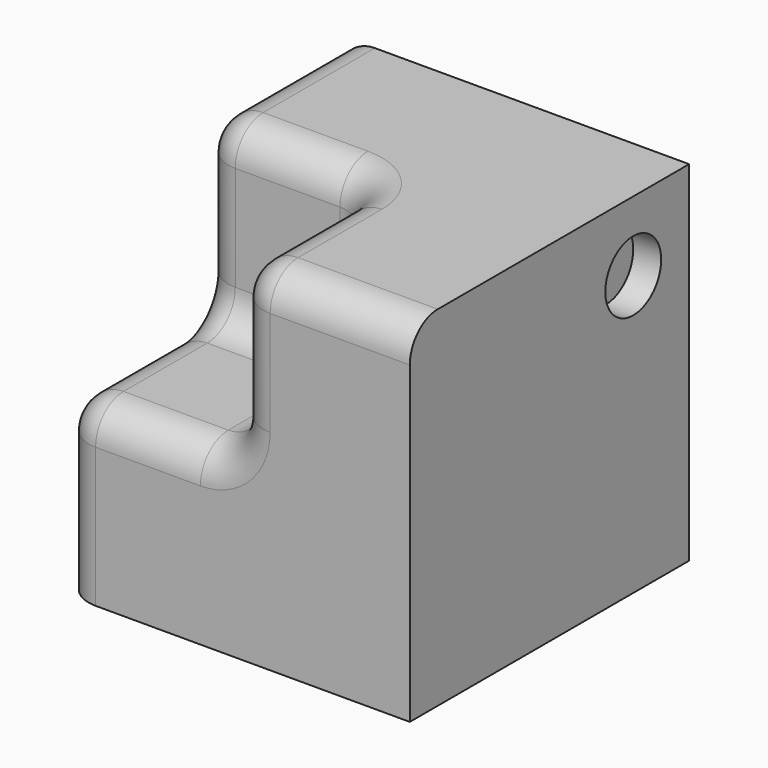
from build123d import *

# Parameters (mm, degrees)
F0_W           = 50
F0_H           = 50
F1_DEPTH       = 50
F3_D           = 2
F3_CBORE_D     = 10
F3_CBORE_DEPTH = 4
F4_W           = 25
F4_H           = 25
F5_DEPTH       = 25
F6_R           = 5


with BuildPart() as f1:
    # F0 (on Top) → F1 (new body)
    with BuildSketch(Plane.XY):
        Rectangle(F0_W, F0_H)
    extrude(amount=F1_DEPTH)

    # F3 (through all)
    with Locations(Plane.YZ.offset(25)):
        with Locations((15, 40)):
            CounterBoreHole(F3_D / 2, F3_CBORE_D / 2, F3_CBORE_DEPTH)

    # F4 (on face) → F5 (cut)
    with BuildSketch(Plane.XZ.offset(25)):
        with Locations((-12.5, 37.5)):
            Rectangle(F4_W, F4_H)
    extrude(amount=-F5_DEPTH, mode=Mode.SUBTRACT)

    # F6
    f6_edges = [f1.edges().sort_by_distance(p)[0] for p in [
        (-12.5, 0, 25),
        (-25, 0, 37.5),
        (0, 0, 37.5),
        (0, -12.5, 50),
        (0, -25, 37.5),
        (-12.5, -25, 25),
        (0, -12.5, 25),
        (-25, 12.5, 50),
        (12.5, -25, 50),
        (-25, -25, 12.5),
        (-12.5, 0, 50),
        (-25, -12.5, 25),
    ]]
    fillet(f6_edges, radius=F6_R)


solid = f1.part
